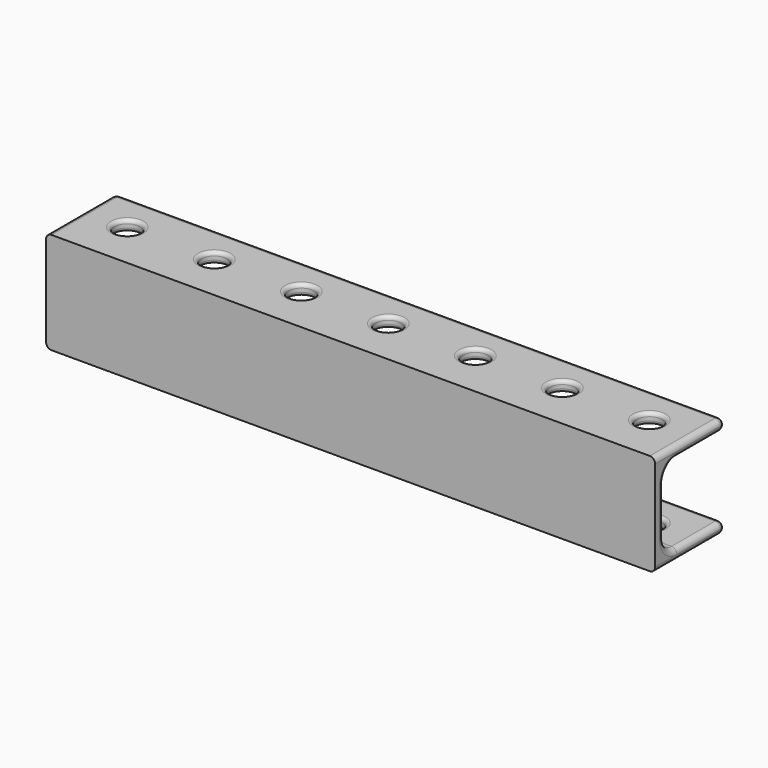
from build123d import *

# Parameters (mm, degrees)
F1_DEPTH = 168
F2_R     = 3.5
F3_DEPTH = 28.001
F4_R     = 4.5
F5_R     = 1.49999
F6_R     = 1


# Not quite as in the source:
# - a fillet or chamfer is up to 0.001 mm smaller than in the source, because OpenCascade refuses the exact size


with BuildPart() as f1:
    # F0 (on Right) → F1 (new body)
    with BuildSketch(Plane.YZ):
        Polygon((24, 28), (0, 28), (0, 0), (24, 0), (24, 3), (3, 3), (3, 25), (24, 25), align=None)
    extrude(amount=F1_DEPTH)

    # F2 (on face) → F3 (cut, through all)
    with BuildSketch(Plane.XY.offset(28)):
        with Locations((12, 13)):
            Circle(F2_R)
        with Locations((36, 13)):
            Circle(F2_R)
        with Locations((60, 13)):
            Circle(F2_R)
        with Locations((84, 13)):
            Circle(F2_R)
        with Locations((108, 13)):
            Circle(F2_R)
        with Locations((132, 13)):
            Circle(F2_R)
        with Locations((156, 13)):
            Circle(F2_R)
    extrude(amount=-F3_DEPTH, mode=Mode.SUBTRACT)

    # F4
    f4_edges = [f1.edges().sort_by_distance(p)[0] for p in [
        (84, 3, 3),
        (84, 3, 25),
    ]]
    fillet(f4_edges, radius=F4_R)

    # F5 (radius 1.5 in the source; OpenCascade refuses exactly that, so slightly less here)
    f5_edges = [f1.edges().sort_by_distance(p)[0] for p in [
        (84, 24, 3),
        (84, 24, 25),
        (84, 24, 28),
        (84, 24, 0),
        (0, 24, 1.5),
        (0, 24, 26.5),
        (168, 24, 1.5),
        (168, 24, 26.5),
        (168, 12, 0),
        (168, 15.75, 3),
        (168, 12, 28),
        (0, 15.75, 25),
        (0, 12, 28),
        (0, 12, 0),
    ]]
    fillet(f5_edges, radius=F5_R)

    # F6
    f6_edges = [f1.edges().sort_by_distance(p)[0] for p in [
        (8.5, 13, 28),
        (32.5, 13, 28),
        (8.5, 13, 25),
        (32.5, 13, 25),
        (56.5, 13, 28),
        (56.5, 13, 25),
        (80.5, 13, 28),
        (80.5, 13, 25),
        (104.5, 13, 28),
        (104.5, 13, 25),
        (128.5, 13, 28),
        (8.5, 13, 0),
        (32.5, 13, 0),
        (32.5, 13, 3),
        (8.5, 13, 3),
        (56.5, 13, 0),
        (80.5, 13, 0),
        (104.5, 13, 0),
        (128.5, 13, 0),
        (152.5, 13, 0),
        (56.5, 13, 3),
        (80.5, 13, 3),
        (104.5, 13, 3),
        (128.5, 13, 3),
        (152.5, 13, 3),
        (128.5, 13, 25),
        (152.5, 13, 25),
        (152.5, 13, 28),
    ]]
    fillet(f6_edges, radius=F6_R)


solid = f1.part
